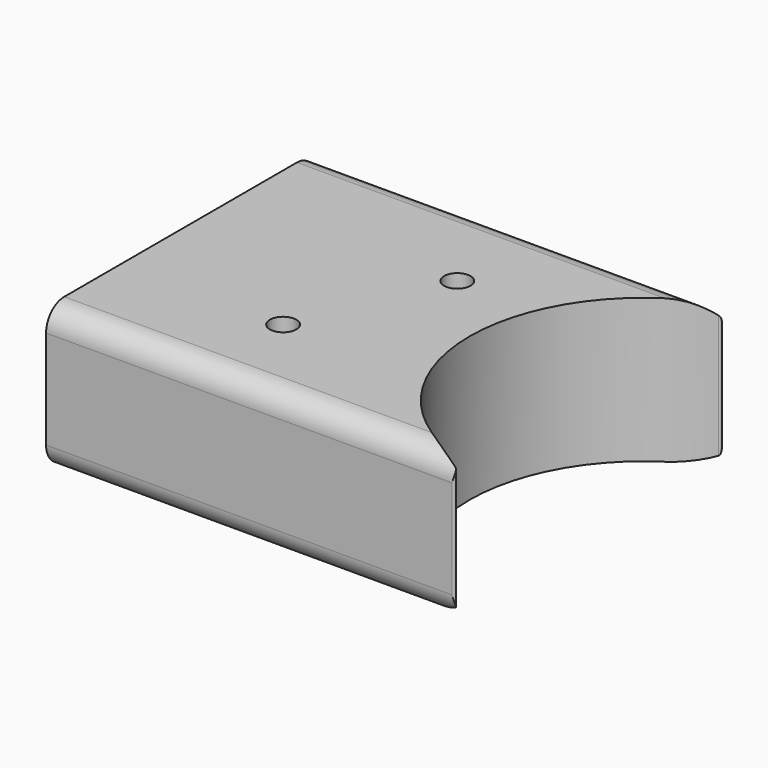
from build123d import *

# Parameters (mm, degrees)
F0_R         = 3.5
F1_DEPTH     = 19.05
F2_F1_R      = 0.5
F2_F2_R      = 0.5
F3_T3_DEPTH  = 137.4526696533
F3_T6_DEPTH  = 137.4526696533
F3_T9_DEPTH  = 137.4526696533
F3_T12_DEPTH = 137.4526696533
F3_T15_ANGLE = 359.64
F3_S16_R     = 6
F3_T17_DEPTH = 5
F3_T20_ANGLE = 359.64
F3_S21_R     = 6
F3_T22_DEPTH = 5
F3_T25_ANGLE = 359.64
F3_S26_R     = 6
F3_T27_DEPTH = 5
F3_T30_ANGLE = 359.64
F3_S31_R     = 6
F3_T32_DEPTH = 5


# Not quite as in the source:
# - a fillet or chamfer that OpenCascade refuses, or shapes differently, is made with other operations: its cross-section is extruded or revolved along the edge and cut away or added


with BuildPart() as f1:
    # F0 (on Top) → F1 (new body, symmetric)
    with BuildSketch(Plane.XY):
        with BuildLine():
            Line((54.843098412, 44.5), (-56, 44.5))
            Line((-56, 44.5), (-56, -44.5))
            Line((-56, -44.5), (54.843098412, -44.5))
            ThreePointArc((54.843098412, -44.5), (20.4942786098, 0), (54.843098412, 44.5))
        make_face()
        with Locations((-12.8994788975, -19.9518427253)):
            Circle(F0_R, mode=Mode.SUBTRACT)
        with Locations((3.0200458132, 17.7928358316)):
            Circle(F0_R, mode=Mode.SUBTRACT)
    extrude(amount=F1_DEPTH, both=True)

    # F2: fillet of radius 0.5 on 2 edges, made by hand

    # F2_f1
    f2_f1_edges = [f1.edges().sort_by_distance(p)[0] for p in [
        (54.843098412, 44.5, 0),
    ]]
    fillet(f2_f1_edges, radius=F2_F1_R)

    # F2_f2
    f2_f2_edges = [f1.edges().sort_by_distance(p)[0] for p in [
        (54.843098412, -44.5, 0),
    ]]
    fillet(f2_f2_edges, radius=F2_F2_R)

    # F3: fillet of radius 6 on 4 edges, made by hand


with BuildPart() as f3_tool1:
    # F3_s2 → F3_t3 (new body)
    with BuildSketch(Plane.YZ.offset(-71)):
        with BuildLine():
            ThreePointArc((-38.5, 19.05), (-42.7426406871, 17.2926406871), (-44.5, 13.05))
            Line((-44.5, 13.05), (-44.5, 19.05))
            Line((-44.5, 19.05), (-38.5, 19.05))
        make_face()
    extrude(amount=F3_T3_DEPTH)


with BuildPart() as f3_tool4:
    # F3_s5 → F3_t6 (new body)
    with BuildSketch(Plane.YZ.offset(-71)):
        with BuildLine():
            ThreePointArc((-38.5, -19.05), (-42.7426406871, -17.2926406871), (-44.5, -13.05))
            Line((-44.5, -13.05), (-44.5, -19.05))
            Line((-44.5, -19.05), (-38.5, -19.05))
        make_face()
    extrude(amount=F3_T6_DEPTH)


with BuildPart() as f3_tool7:
    # F3_s8 → F3_t9 (new body)
    with BuildSketch(Plane.YZ.offset(66.4526696533)):
        with BuildLine():
            ThreePointArc((38.5, 19.05), (42.7426406871, 17.2926406871), (44.5, 13.05))
            Line((44.5, 13.05), (44.5, 19.05))
            Line((44.5, 19.05), (38.5, 19.05))
        make_face()
    extrude(amount=-F3_T9_DEPTH)


with BuildPart() as f3_tool10:
    # F3_s11 → F3_t12 (new body)
    with BuildSketch(Plane.YZ.offset(66.4526696533)):
        with BuildLine():
            ThreePointArc((38.5, -19.05), (42.7426406871, -17.2926406871), (44.5, -13.05))
            Line((44.5, -13.05), (44.5, -19.05))
            Line((44.5, -19.05), (38.5, -19.05))
        make_face()
    extrude(amount=-F3_T12_DEPTH)


with BuildPart() as f3_tool13:
    # F3_s14 → F3_t15 (revolve)
    with BuildSketch(Plane(origin=(51.7270912874, 0.325015177, 0), x_dir=(0, 0, 1), z_dir=(0.9999802609, 0.006283144, 0))):
        with BuildLine():
            ThreePointArc((-15.4479157617, -43.6758469468), (-14.2747448714, -44.0495170091), (-13.05, -44.1758469468))
            Line((-13.05, -44.1758469468), (-19.05, -44.1758469468))
            Line((-19.05, -44.1758469468), (-19.05, -43.6758469468))
            Line((-19.05, -43.6758469468), (-15.4479157617, -43.6758469468))
        make_face()
    revolve(axis=Axis((51.4526696533, 44, -19.05), (0, 0, 1)), revolution_arc=F3_T15_ANGLE)

    # F3_s16 → F3_t17 (cut, symmetric)
    with BuildSketch(Plane.YZ.offset(51.5)):
        with Locations((38.5, -13.05)):
            Circle(F3_S16_R)
    extrude(amount=F3_T17_DEPTH, both=True, mode=Mode.SUBTRACT)


with BuildPart() as f3_tool18:
    # F3_s19 → F3_t20 (revolve)
    with BuildSketch(Plane(origin=(51.7270912874, -0.325015177, 0), x_dir=(0, 0, 1), z_dir=(0.9999802609, -0.006283144, 0))):
        with BuildLine():
            ThreePointArc((-15.4479157617, 43.6758469468), (-14.2747448714, 44.0495170091), (-13.05, 44.1758469468))
            Line((-13.05, 44.1758469468), (-19.05, 44.1758469468))
            Line((-19.05, 44.1758469468), (-19.05, 43.6758469468))
            Line((-19.05, 43.6758469468), (-15.4479157617, 43.6758469468))
        make_face()
    revolve(axis=Axis((51.4526696533, -44, -19.05), (0, 0, -1)), revolution_arc=F3_T20_ANGLE)

    # F3_s21 → F3_t22 (cut, symmetric)
    with BuildSketch(Plane.YZ.offset(51.5)):
        with Locations((-38.5, -13.05)):
            Circle(F3_S21_R)
    extrude(amount=F3_T22_DEPTH, both=True, mode=Mode.SUBTRACT)


with BuildPart() as f3_tool23:
    # F3_s24 → F3_t25 (revolve)
    with BuildSketch(Plane(origin=(51.7270912874, 0.325015177, 0), x_dir=(0, 0, 1), z_dir=(0.9999802609, 0.006283144, 0))):
        with BuildLine():
            ThreePointArc((13.05, -44.1758469468), (14.2747448714, -44.0495170091), (15.4479157617, -43.6758469468))
            Line((15.4479157617, -43.6758469468), (19.05, -43.6758469468))
            Line((19.05, -43.6758469468), (19.05, -44.1758469468))
            Line((19.05, -44.1758469468), (13.05, -44.1758469468))
        make_face()
    revolve(axis=Axis((51.4526696533, 44, 19.05), (0, 0, 1)), revolution_arc=F3_T25_ANGLE)

    # F3_s26 → F3_t27 (cut, symmetric)
    with BuildSketch(Plane.YZ.offset(51.5)):
        with Locations((38.5, 13.05)):
            Circle(F3_S26_R)
    extrude(amount=F3_T27_DEPTH, both=True, mode=Mode.SUBTRACT)


with BuildPart() as f3_tool28:
    # F3_s29 → F3_t30 (revolve)
    with BuildSketch(Plane(origin=(51.7270912874, -0.325015177, 0), x_dir=(0, 0, 1), z_dir=(0.9999802609, -0.006283144, 0))):
        with BuildLine():
            ThreePointArc((13.05, 44.1758469468), (14.2747448714, 44.0495170091), (15.4479157617, 43.6758469468))
            Line((15.4479157617, 43.6758469468), (19.05, 43.6758469468))
            Line((19.05, 43.6758469468), (19.05, 44.1758469468))
            Line((19.05, 44.1758469468), (13.05, 44.1758469468))
        make_face()
    revolve(axis=Axis((51.4526696533, -44, 19.05), (0, 0, -1)), revolution_arc=F3_T30_ANGLE)

    # F3_s31 → F3_t32 (cut, symmetric)
    with BuildSketch(Plane.YZ.offset(51.5)):
        with Locations((-38.5, 13.05)):
            Circle(F3_S31_R)
    extrude(amount=F3_T32_DEPTH, both=True, mode=Mode.SUBTRACT)


with BuildPart() as f1_1:
    add(f1.part)

    # F3_t33: cut F3_tool1, F3_tool4, F3_tool7, F3_tool10, F3_tool13, F3_tool18, F3_tool23, F3_tool28
    add([f3_tool1.part, f3_tool4.part, f3_tool7.part, f3_tool10.part, f3_tool13.part, f3_tool18.part, f3_tool23.part, f3_tool28.part], mode=Mode.SUBTRACT)


solid = f1_1.part
